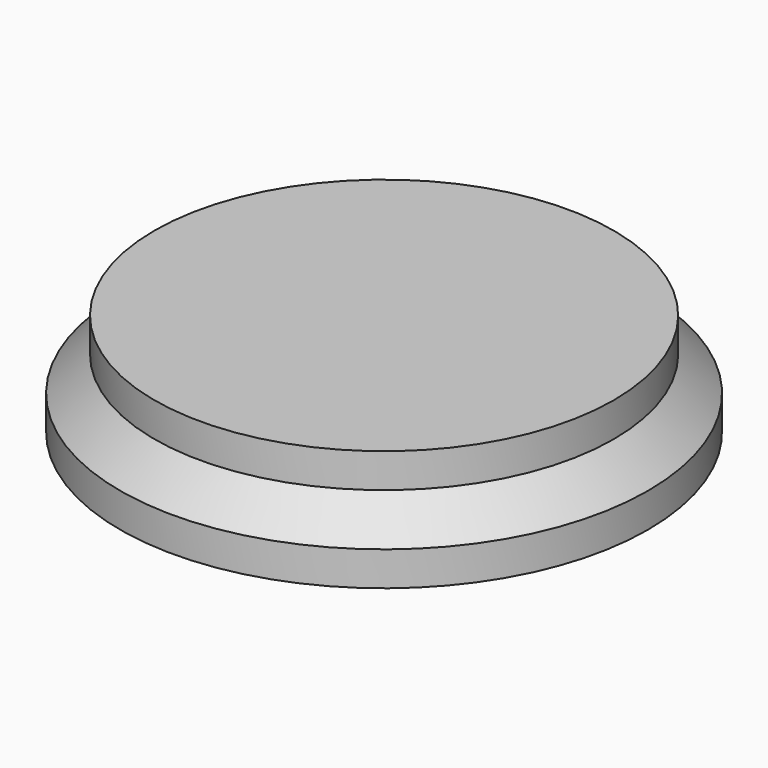
from build123d import *

# Parameters (mm, degrees)
F0_R     = 19.25
F1_DEPTH = 5
F2_R     = 16.75
F3_DEPTH = 2.5
F4_R     = 16.75
F5_DEPTH = 2.5
F6_SIZE  = 2.49999


# Not quite as in the source:
# - a fillet or chamfer is up to 0.001 mm smaller than in the source, because OpenCascade refuses the exact size


with BuildPart() as f1:
    # F0 (on Top) → F1 (new body)
    with BuildSketch(Plane.XY):
        Circle(F0_R)
    extrude(amount=F1_DEPTH)

    # F2 (on face) → F3 (join)
    with BuildSketch(Plane.XY.offset(5)):
        Circle(F2_R)
    extrude(amount=F3_DEPTH)

    # F4 (on face) → F5 (cut)
    with BuildSketch(Plane(origin=(0, 0, 0), x_dir=(1, 0, 0), z_dir=(0, 0, -1))):
        Circle(F4_R)
    extrude(amount=-F5_DEPTH, mode=Mode.SUBTRACT)

    # F6 (size 2.5 in the source; OpenCascade refuses exactly that, so slightly less here)
    f6_edges = [f1.edges().sort_by_distance(p)[0] for p in [
        (-19.25, 0, 5),
    ]]
    chamfer(f6_edges, length=F6_SIZE)


solid = f1.part
